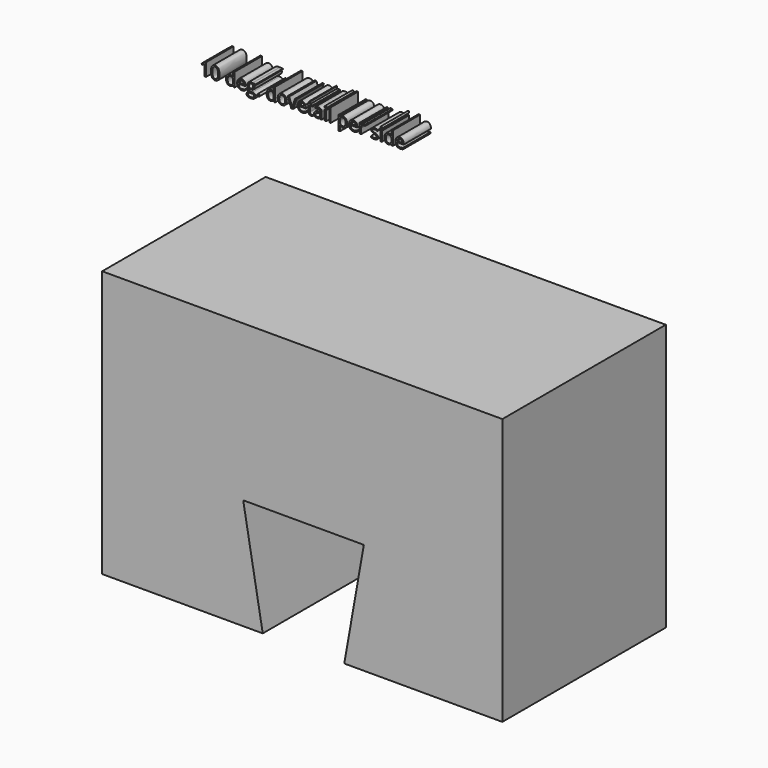
from build123d import *

# Parameters (mm, degrees)
F1_DEPTH     = 152.4
F2_TEXT_SIZE = 13.4609018763
F3_DEPTH     = 25.4


# Not quite as in the source:
# - Text() gives the source's letters only with a copy of the font that has no kerning and outlines rounded to 1/6400 em; it was checked with that copy


with BuildPart() as f1:
    # F0 (on Front) → F1 (new body)
    with BuildSketch(Plane.XZ):
        Polygon((31.3360956165, -99.4378179312), (149.2467522621, -99.4378179312), (149.2467522621, 99.4378179312), (-149.2467522621, 99.4378179312), (-149.2467522621, -99.4378179312), (-29.486478235, -99.4378179312), (-44.0660607886, -16.7528964576), (45.9156781701, -16.7528964576), align=None)
    extrude(amount=F1_DEPTH)


with BuildPart() as f3:
    # F2 (on Front) → F3 (new body)
    with BuildSketch(Plane.XZ):
        with Locations((-178.0739724636, 167.6046401262)):
            Text('10 deg. dovetail per side', F2_TEXT_SIZE, font='Open Sans', text_align=(TextAlign.LEFT, TextAlign.BOTTOM))
    extrude(amount=F3_DEPTH)


solid = Compound([f1.part, f3.part])
